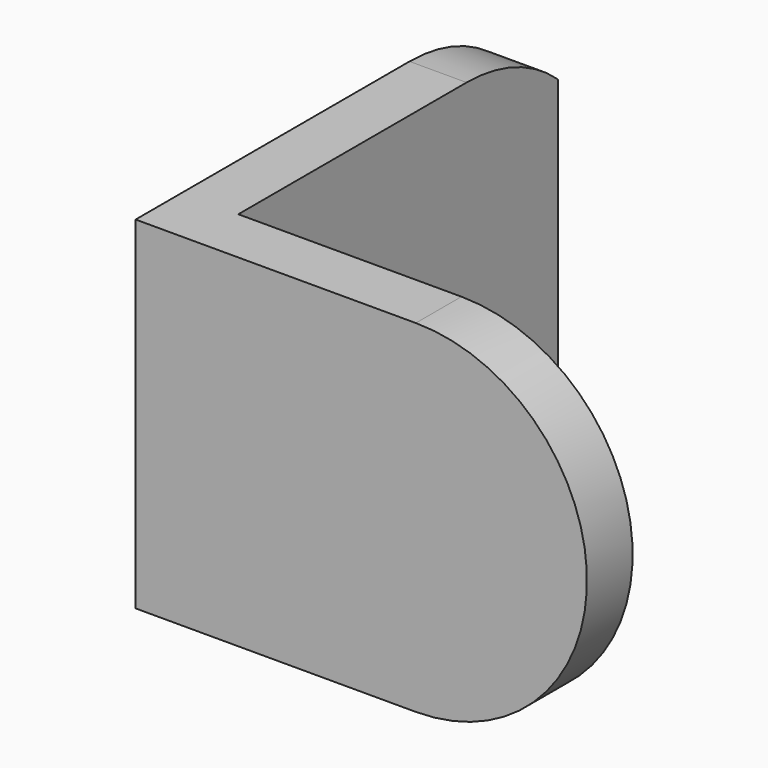
from build123d import *

# Parameters (mm, degrees)
F1_DEPTH = 30
F3_DEPTH = 15.3
F5_DEPTH = 25


with BuildPart() as f1:
    # F0 (on Top) → F1 (new body)
    with BuildSketch(Plane.XY):
        Polygon((4.9999998882, 40), (0, 40), (0, 0), (40, 0), (40, 4.9999998882), (4.9999998882, 4.9999998882), align=None)
    extrude(amount=-F1_DEPTH)

    # F2 (on face) → F3 (cut)
    with BuildSketch(Plane.YZ.offset(4.9999998882)):
        with BuildLine():
            Line((40, -3.8196602917), (40, 0))
            Line((40, 0), (29.9999997997, 0))
            ThreePointArc((29.9999997997, 0), (35.3523312718, -0.9874146635), (40, -3.8196602917))
        make_face()
        with BuildLine():
            Line((40, -30), (40, -26.1803397083))
            ThreePointArc((40, -26.1803397083), (35.3523313132, -29.0125853207), (29.9999998882, -30))
            Line((29.9999998882, -30), (40, -30))
        make_face()
    extrude(amount=-F3_DEPTH, mode=Mode.SUBTRACT)

    # F4 (on face) → F5 (cut)
    with BuildSketch(Plane(origin=(0, 4.9999998882, 0), x_dir=(-1, 0, 0), z_dir=(0, 1, 0))):
        with BuildLine():
            Line((-24.5546065271, 0), (-40, 0))
            Line((-40, 0), (-40, -30))
            Line((-40, -30), (-24.5546074611, -30))
            ThreePointArc((-24.5546074611, -30), (-39.5546074611, -14.999999533), (-24.5546065271, 0))
        make_face()
    extrude(amount=-F5_DEPTH, mode=Mode.SUBTRACT)


solid = f1.part
